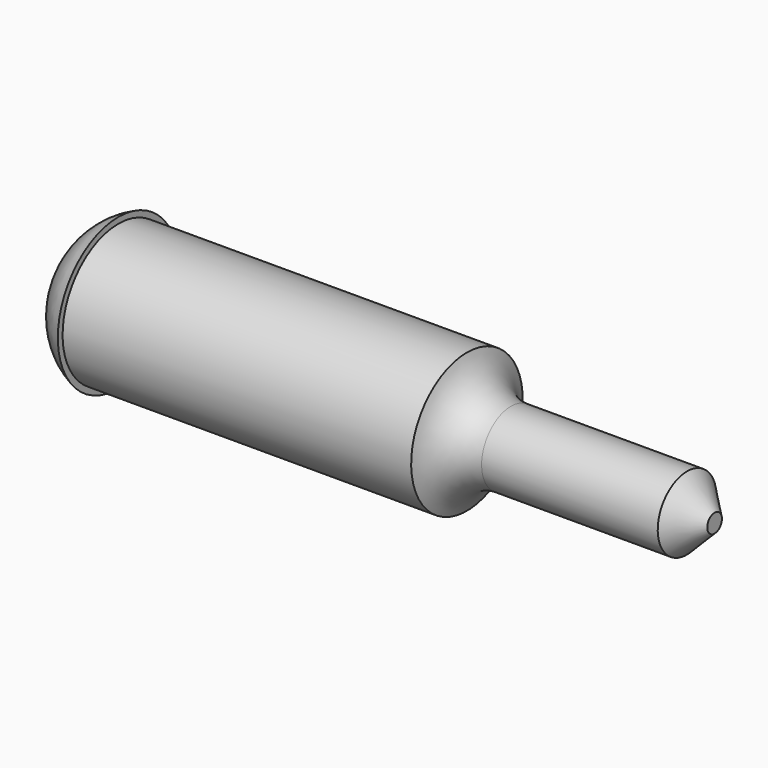
from build123d import *

# Parameters (mm, degrees)
F3_SIZE = 3


# Not quite as in the source:
# - a fillet or chamfer that OpenCascade refuses, or shapes differently, is made with other operations: its cross-section is extruded or revolved along the edge and cut away or added


with BuildPart() as f1:
    # F0 (on Front) → F1 (revolve)
    with BuildSketch(Plane.XZ):
        Polygon((0, 8.25), (0, 0), (70, 0), (70, 4), (43, 4), (43, 7.6), (5, 7.6), (5, 8.25), align=None)
    revolve(axis=Axis((35, 0, 0), (1, 0, 0)))

    # F2: fillet of radius 5 on 1 edges, made by hand

    # F2_s1 → F2_t2 (revolve)
    with BuildSketch(Plane.XZ):
        with BuildLine():
            ThreePointArc((47.8, 4), (44.8, 5), (43, 7.6))
            Line((43, 7.6), (43, 4))
            Line((43, 4), (47.8, 4))
        make_face()
    revolve(axis=Axis((43, 0, 0), (1, 0, 0)))

    # F3
    f3_edges = [f1.edges().sort_by_distance(p)[0] for p in [
        (70, 0, -4),
    ]]
    chamfer(f3_edges, length=F3_SIZE)

    # F4: fillet of radius 8.1 on 1 edges, made by hand

    # F4_s1 → F4_t2 (revolve, cut)
    with BuildSketch(Plane.XZ):
        with BuildLine():
            ThreePointArc((5, 8.25), (1.3650167038, 5.2666852265), (0, 0.7666852265))
            Line((0, 0.7666852265), (0, 8.25))
            Line((0, 8.25), (5, 8.25))
        make_face()
    revolve(axis=Axis((0, 0, 0), (1, 0, 0)), mode=Mode.SUBTRACT)


solid = f1.part
